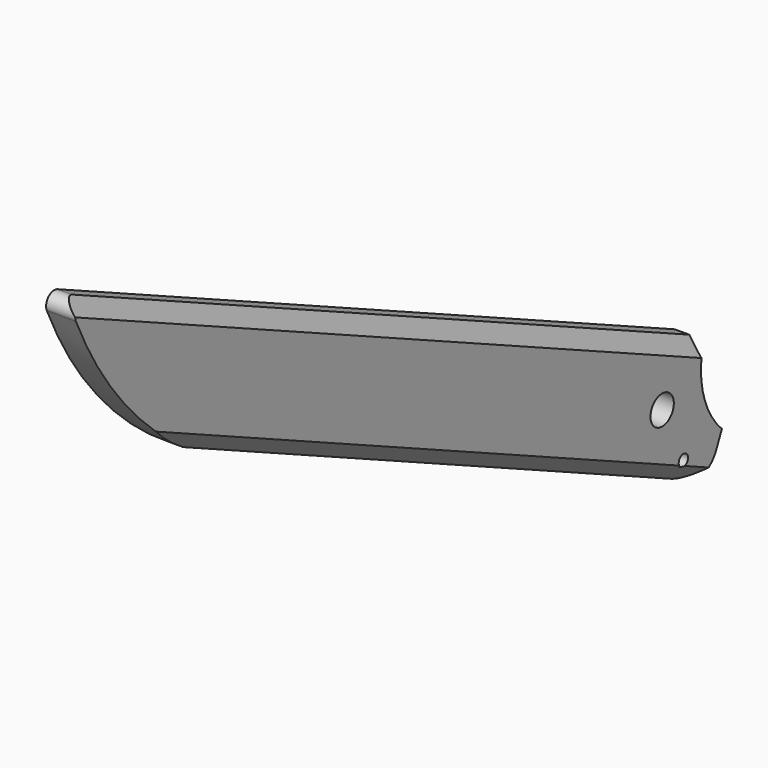
from build123d import *

# Parameters (mm, degrees)
F0_R        = 1
F0_R_2      = 2.5
F1_DEPTH    = 5
F2_T1_DEPTH = 140.5508565822
F2_T3_DEPTH = 158.1494237613


# Not quite as in the source:
# - a fillet or chamfer that OpenCascade refuses, or shapes differently, is made with other operations: its cross-section is extruded or revolved along the edge and cut away or added


with BuildPart() as f1:
    # F0 (on Right) → F1 (new body)
    with BuildSketch(Plane.YZ):
        with BuildLine():
            Line((-238.351838073, 51.1362271676), (-133.7205907933, 3.81650843))
            ThreePointArc((-133.7205907933, 3.81650843), (-129.8957188572, 3.6939702207), (-127.1044783752, 6.3119155052))
            Line((-127.1044783752, 6.3119155052), (-125.8958157643, 8.9844562534))
            ThreePointArc((-125.8958157643, 8.9844562534), (-129.9178817918, 15.9435567205), (-129.7697865993, 23.9799839275))
            Line((-129.7697865993, 23.9799839275), (-224.5101433949, 66.8265250251))
            Line((-224.5101433949, 66.8265250251), (-262.1519725075, 83.8501275596))
            ThreePointArc((-262.1519725075, 83.8501275596), (-264.0478442183, 83.5411975558), (-264.4983908426, 81.6739067294))
            ThreePointArc((-264.4983908426, 81.6739067294), (-264.4532671282, 81.571051598), (-264.4079761186, 81.4682700232))
            ThreePointArc((-264.4079761186, 81.4682700232), (-253.6243159552, 64.3742338109), (-238.351838073, 51.1362271676))
        make_face()
        with Locations((-134.1624917959, 7.5852589493)):
            Circle(F0_R, mode=Mode.SUBTRACT)
        with Locations((-138.7114049438, 17.0487332662)):
            Circle(F0_R_2, mode=Mode.SUBTRACT)
        with BuildLine():
            ThreePointArc((-264.4983908426, 81.6739067294), (-264.4565130864, 81.5696244091), (-264.4079761186, 81.4682700232))
            ThreePointArc((-264.4079761186, 81.4682700232), (-264.4532671282, 81.571051598), (-264.4983908426, 81.6739067294))
        make_face()
    extrude(amount=F1_DEPTH)

    # F2: chamfer of 2.5 on 2 edges, made by hand

    # F2_s2 → F2_t1 (cut)
    with BuildSketch(Plane(origin=(0, -234.652694271, 106.1222128437), x_dir=(1, 0, 0), z_dir=(0, 0.9111519493, -0.4120705343))):
        Polygon((2.5, 51.6248961977), (5, 49.1248961977), (5, 51.6248961977), align=None)
    extrude(amount=F2_T1_DEPTH, mode=Mode.SUBTRACT)

    # F2_s4 → F2_t3 (cut)
    with BuildSketch(Plane(origin=(0, -110.8801138075, 50.1457827883), x_dir=(1, 0, 0), z_dir=(0, -0.9111519493, 0.4120705343))):
        Polygon((2.5, -31.6248961977), (5, -34.1248961977), (5, -31.6248961977), align=None)
    extrude(amount=F2_T3_DEPTH, mode=Mode.SUBTRACT)


solid = f1.part
